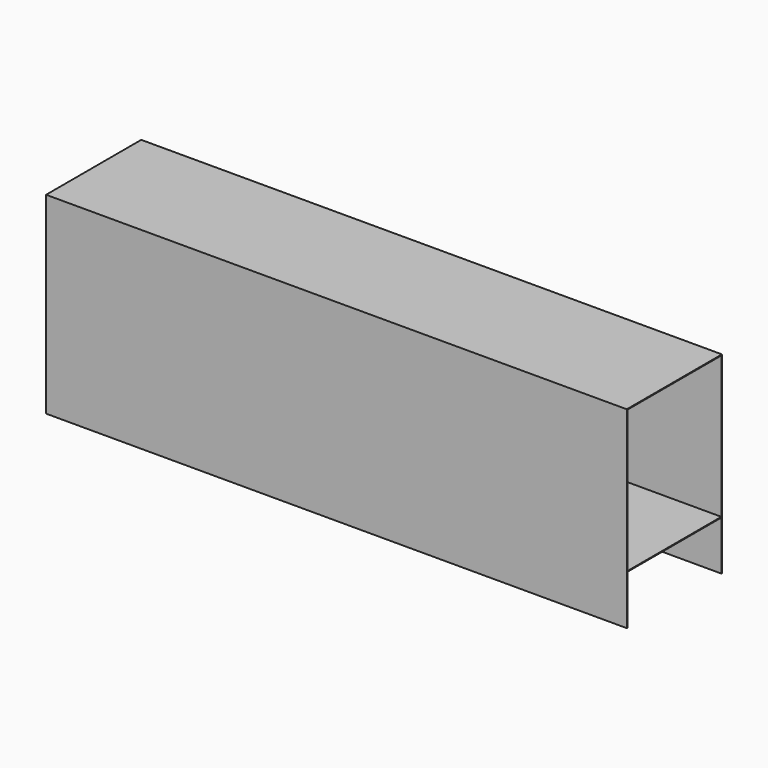
from build123d import *

# Parameters (mm, degrees)
F1_DEPTH = 101.6


# Not quite as in the source:
# - ends of sketch curves that miss each other by under 0.0002 mm in the source are joined


with BuildPart() as f1:
    # F0 (on Right) → F1 (new body, symmetric)
    with BuildSketch(Plane.YZ):
        Polygon((-20.8060556405, -33.7167573632), (-20.5520556405, -33.7167573632), (-20.5520556405, -16.4791475981), (20.5520556405, -16.4791475981), (20.5520556405, -33.7184855556), (20.8060556405, -33.7167573632), (20.8060556405, 33.7167573632), (-20.8060556405, 33.7167573632), align=None)
        Polygon((20.5520556405, -16.2251475981), (-20.5520556405, -16.2251475981), (-20.5520556405, 33.4627573632), (20.5521062016, 33.4627573632), align=None, mode=Mode.SUBTRACT)
    extrude(amount=F1_DEPTH, both=True)


solid = f1.part
